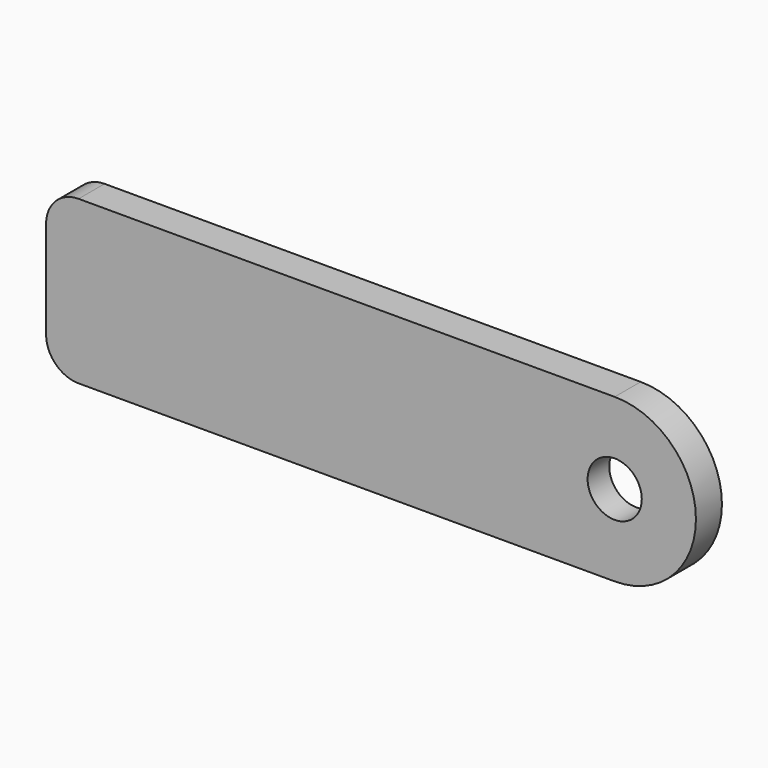
from build123d import *

# Parameters (mm, degrees)
F0_R         = 2.5
F1_DEPTH     = 3
F2_TEXT_SIZE = 9.7222222222
F3_DEPTH     = 1
F5_DEPTH     = 0.5


# Not quite as in the source:
# - a feature names something its author has since deleted; it is built from what else it names
# - Text() gives the source's letters only with a copy of the font that has no kerning and outlines rounded to 1/6400 em; it was checked with that copy


with BuildPart() as f1:
    # F0 (on Front) → F1 (new body)
    with BuildSketch(Plane.XZ):
        with BuildLine():
            Line((52.5, 7.5), (3, 7.5))
            ThreePointArc((3, 7.5), (0.8786796564, 6.6213203436), (0, 4.5))
            Line((0, 4.5), (0, -4.5))
            ThreePointArc((0, -4.5), (0.8786796564, -6.6213203436), (3, -7.5))
            Line((3, -7.5), (52.5, -7.5))
            ThreePointArc((52.5, -7.5), (60, 0), (52.5, 7.5))
        make_face()
        with Locations((52.5, 0)):
            Circle(F0_R, mode=Mode.SUBTRACT)
    extrude(amount=F1_DEPTH)

    # F2 (on face) → F3 (cut)
    with BuildSketch(Plane(origin=(0, 0, 0), x_dir=(-1, 0, 0), z_dir=(0, 1, 0))):
        with Locations((-37.6666666667, -3.5)):
            Text('guido', F2_TEXT_SIZE, font='Open Sans', text_align=(TextAlign.LEFT, TextAlign.BOTTOM))
    extrude(amount=-F3_DEPTH, mode=Mode.SUBTRACT)

    # F4 (on face) → F5 (cut)
    with BuildSketch(Plane(origin=(0, 0, 0), x_dir=(-1, 0, 0), z_dir=(0, 1, 0))):
        with BuildLine():
            ThreePointArc((-2.5999999419, 4.5), (-2.7171572464, 4.7828427536), (-3, 4.9000000581))
            Line((-3, 4.9000000581), (-52.5, 4.9000000581))
            ThreePointArc((-52.5, 4.9000000581), (-57.4000000581, 0), (-52.5, -4.9000000581))
            Line((-52.5, -4.9000000581), (-3, -4.9000000581))
            ThreePointArc((-3, -4.9000000581), (-2.7171572464, -4.7828427536), (-2.5999999419, -4.5))
            Line((-2.5999999419, -4.5), (-2.5999999419, 4.5))
        make_face()
    extrude(amount=-F5_DEPTH, mode=Mode.SUBTRACT)


solid = f1.part
